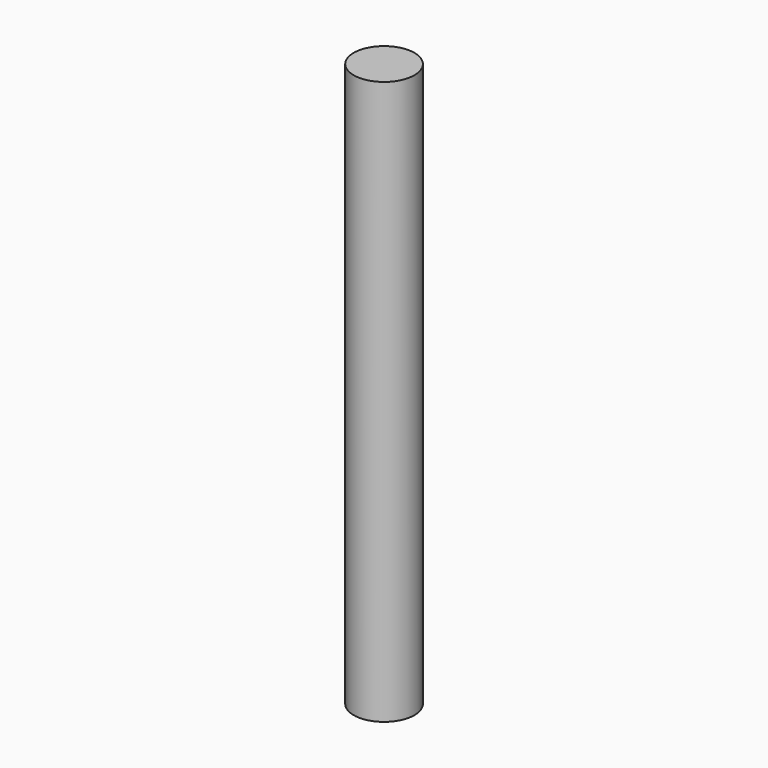
from build123d import *

# Parameters (mm, degrees)
F2_R          = 8.20995575
F3_DEPTH      = 76.2
F3_DEPTH_BACK = 76.2


# Not quite as in the source:
# - the program builds the solid bodies; features that only make, move or delete a surface that nothing else refers to are left out


with BuildPart() as f3:
    # F2 (on Top) → F3 (new body, two sides)
    with BuildSketch(Plane.XY) as f3_sk:
        Circle(F2_R)
    extrude(amount=F3_DEPTH)
    extrude(f3_sk.sketch, amount=-F3_DEPTH_BACK)


solid = f3.part
